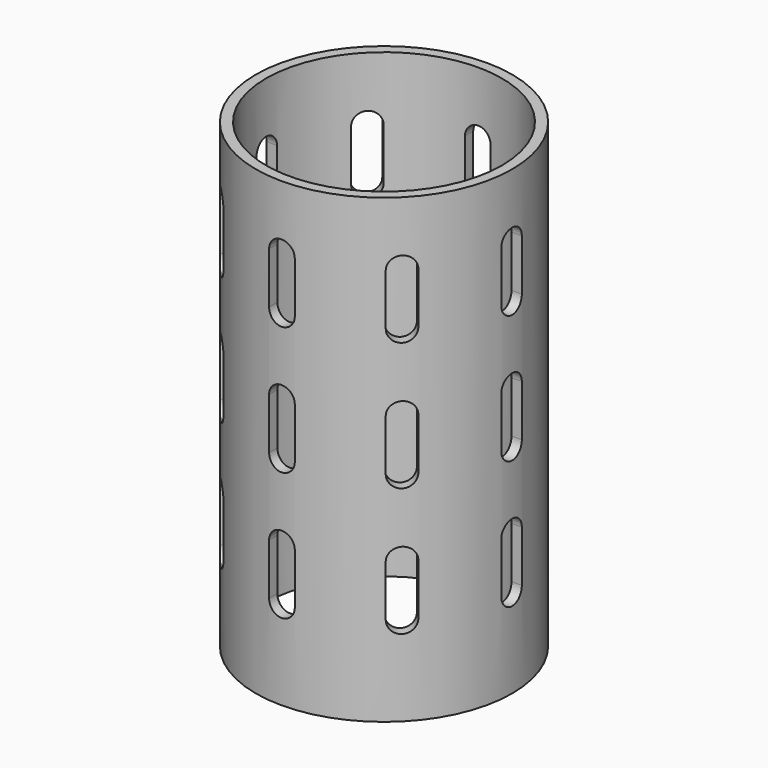
from build123d import *

# Parameters (mm, degrees)
F0_W            = 25
F0_H            = 90
F2_T            = -2
F4_DEPTH        = 84.2
F4_COPIES_COUNT = 8


# Not quite as in the source:
# - a pattern or mirror of a feature is missing from the dataset's text; its kind, count and spacing are read off the source's solid


with BuildPart() as f1:
    # F0 (on Front) → F1 (revolve)
    with BuildSketch(Plane.XZ):
        with Locations((12.5, 0)):
            Rectangle(F0_W, F0_H)
    revolve(axis=Axis((0, 0, 3.7005562335), (0, 0, -1)))

    # F2
    f2_openings = [f1.faces().sort_by_distance(p)[0] for p in [
        (0, 0, 45),
        (0, 0, -45),
    ]]
    offset(amount=F2_T, openings=f2_openings)

    # F3 (on Front) → F4 (cut)
    with BuildSketch(Plane.XZ):
        with BuildLine():
            ThreePointArc((2.5, 32.5), (0, 35), (-2.5, 32.5))
            Line((-2.5, 32.5), (-2.5, 22.5))
            ThreePointArc((-2.5, 22.5), (0, 20), (2.5, 22.5))
            Line((2.5, 22.5), (2.5, 32.5))
        make_face()
        with BuildLine():
            Line((-2.5, 7.5), (-2.5, -2.5))
            ThreePointArc((-2.5, -2.5), (0, -5), (2.5, -2.5))
            Line((2.5, -2.5), (2.5, 7.5))
            ThreePointArc((2.5, 7.5), (0, 10), (-2.5, 7.5))
        make_face()
        with BuildLine():
            Line((-2.5, -17.5), (-2.5, -27.5))
            ThreePointArc((-2.5, -27.5), (0, -30), (2.5, -27.5))
            Line((2.5, -27.5), (2.5, -17.5))
            ThreePointArc((2.5, -17.5), (0, -15), (-2.5, -17.5))
        make_face()
    f4 = extrude(amount=F4_DEPTH, mode=Mode.SUBTRACT)

    # F4_copies: F4 ×8 about axis
    f4_copies_axis = Axis((0, 0, 0), (0, 0, 1))
    for i in range(1, F4_COPIES_COUNT):
        add(f4.rotate(f4_copies_axis, i * 360 / F4_COPIES_COUNT), mode=Mode.SUBTRACT)


solid = f1.part
